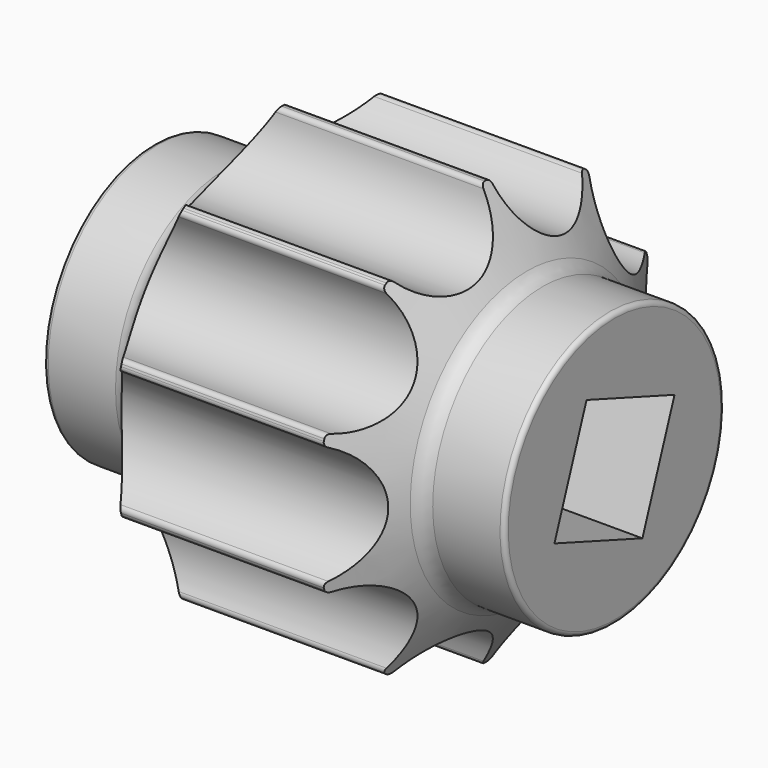
from build123d import *

# Parameters (mm, degrees)
F3_R        = 0.5
F2_R        = 5
F4_DEPTH    = 50
F2_R_2      = 7
F5_DEPTH    = 50
F6_R        = 2
F7_T1_DEPTH = 24.3069691613


# Not quite as in the source:
# - a fillet or chamfer that OpenCascade refuses, or shapes differently, is made with other operations: its cross-section is extruded or revolved along the edge and cut away or added
# - two fillets or chamfers of one size are made in one step


with BuildPart() as f1:
    # F0 (on Front) → F1 (revolve)
    with BuildSketch(Plane.XZ):
        Polygon((-25, 5), (25, 5), (25, 14.9), (16.1, 14.9), (11, 23), (-11, 23), (-16.1, 14.9), (-25, 14.9), align=None)
    revolve(axis=Axis((2.6108596474, 0, 0), (1, 0, 0)))

    # F3
    f3_edges = [f1.edges().sort_by_distance(p)[0] for p in [
        (-25, 0, -14.9),
        (25, 0, -14.9),
    ]]
    fillet(f3_edges, radius=F3_R)

    # F2 (on face) → F4 (cut)
    with BuildSketch(Plane.YZ.offset(25)):
        Polygon((3.7870547807, -8.1426786801), (8.1426786801, 3.7870547807), (-3.7870547807, 8.1426786801), (-8.1426786801, -3.7870547807), align=None)
        Circle(F2_R, mode=Mode.SUBTRACT)
    extrude(amount=-F4_DEPTH, mode=Mode.SUBTRACT)

    # F2 (on face) → F5 (cut)
    with BuildSketch(Plane.YZ.offset(25)):
        with Locations((19.8209163622, 14.4007386812)):
            Circle(F2_R_2)
        with Locations((24.5, 0)):
            Circle(F2_R_2)
        with Locations((19.8209163622, -14.4007386812)):
            Circle(F2_R_2)
        with Locations((7.5709163622, -23.3008846492)):
            Circle(F2_R_2)
        with Locations((-7.5709163622, -23.3008846492)):
            Circle(F2_R_2)
        with Locations((-19.8209163622, -14.4007386812)):
            Circle(F2_R_2)
        with Locations((-24.5, 0)):
            Circle(F2_R_2)
        with Locations((-7.5709163622, 23.3008846492)):
            Circle(F2_R_2)
        with Locations((7.5709163622, 23.3008846492)):
            Circle(F2_R_2)
        with Locations((-19.8209163622, 14.4007386812)):
            Circle(F2_R_2)
    extrude(amount=-F5_DEPTH, mode=Mode.SUBTRACT)

    # F6
    f6_edges = [f1.edges().sort_by_distance(p)[0] for p in [
        (-16.1, 0, -14.9),
        (16.1, 0, -14.9),
    ]]
    fillet(f6_edges, radius=F6_R)

    # F7: fillet of radius 0.5 on 20 edges, made by hand

    # F7_s2 → F7_t1 (cut)
    with BuildSketch(Plane.YZ.offset(-12.1534845806)):
        with BuildLine():
            ThreePointArc((12.7621083082, 18.6049793925), (13.0799593931, 18.7667461577), (13.424750127, 18.6755477571))
            ThreePointArc((13.424750127, 18.6755477571), (13.2367534387, 18.8092625693), (13.0474250079, 18.9410849917))
            ThreePointArc((13.0474250079, 18.9410849917), (12.9074134082, 18.7707853923), (12.7621083082, 18.6049793925))
        make_face()
        with BuildLine():
            ThreePointArc((0.1163605522, 22.9997056551), (0.4489071903, 22.8708238025), (0.6109700008, 22.5531235603))
            ThreePointArc((0.6109700008, 22.5531235603), (0.5908740269, 22.7726716267), (0.5777018563, 22.9927436502))
            ThreePointArc((0.5777018563, 22.9927436502), (0.3470486624, 22.9973815298), (0.1163605522, 22.9997056551))
        make_face()
        with BuildLine():
            ThreePointArc((-12.7621083082, 18.6049793925), (-13.0799593931, 18.7667461577), (-13.424750127, 18.6755477571))
            ThreePointArc((-13.424750127, 18.6755477571), (-13.2367534387, 18.8092625693), (-13.0474250079, 18.9410849917))
            ThreePointArc((-13.0474250079, 18.9410849917), (-12.9074134082, 18.7707853923), (-12.7621083082, 18.6049793925))
        make_face()
        with BuildLine():
            ThreePointArc((-0.1163605522, 22.9997056551), (-0.4489071903, 22.8708238025), (-0.6109700008, 22.5531235603))
            ThreePointArc((-0.6109700008, 22.5531235603), (-0.5908740269, 22.7726716267), (-0.5777018563, 22.9927436502))
            ThreePointArc((-0.5777018563, 22.9927436502), (-0.3470486624, 22.9973815298), (-0.1163605522, 22.9997056551))
        make_face()
        with BuildLine():
            ThreePointArc((13.6130254553, 18.5387577241), (13.8063064847, 18.2390241055), (13.7506785355, 17.8867410805))
            ThreePointArc((13.7506785355, 17.8867410805), (13.8634676667, 18.0761713143), (13.9821662468, 18.261955729))
            ThreePointArc((13.9821662468, 18.261955729), (13.7982899703, 18.4012823981), (13.6130254553, 18.5387577241))
        make_face()
        with BuildLine():
            ThreePointArc((21.2604950115, 7.5503654569), (21.6127260597, 7.4944093388), (21.8380625481, 7.2179653744))
            ThreePointArc((21.8380625481, 7.2179653744), (21.764565627, 7.4366446107), (21.6888789848, 7.6545756502))
            ThreePointArc((21.6888789848, 7.6545756502), (21.4755076282, 7.5990971335), (21.2604950115, 7.5503654569))
        make_face()
        with BuildLine():
            ThreePointArc((21.9099773243, 6.9966344517), (21.8901659611, 6.6405371218), (21.6380952381, 6.3882314559))
            ThreePointArc((21.6380952381, 6.3882314559), (21.8406878598, 6.4751879464), (22.0459183673, 6.5557214203))
            ThreePointArc((22.0459183673, 6.5557214203), (21.9790534962, 6.7765188269), (21.9099773243, 6.9966344517))
        make_face()
        with BuildLine():
            ThreePointArc((21.6380952381, -6.3882314559), (21.8901659611, -6.6405371218), (21.9099773243, -6.9966344517))
            ThreePointArc((21.9099773243, -6.9966344517), (21.9790534962, -6.7765188269), (22.0459183673, -6.5557214203))
            ThreePointArc((22.0459183673, -6.5557214203), (21.8406878598, -6.4751879464), (21.6380952381, -6.3882314559))
        make_face()
        with BuildLine():
            ThreePointArc((21.8380625481, -7.2179653744), (21.6127260597, -7.4944093388), (21.2604950115, -7.5503654569))
            ThreePointArc((21.2604950115, -7.5503654569), (21.4755076282, -7.5990971335), (21.6888789848, -7.6545756502))
            ThreePointArc((21.6888789848, -7.6545756502), (21.764565627, -7.4366446107), (21.8380625481, -7.2179653744))
        make_face()
        with BuildLine():
            ThreePointArc((13.7506785355, -17.8867410805), (13.8063064847, -18.2390241055), (13.6130254553, -18.5387577241))
            ThreePointArc((13.6130254553, -18.5387577241), (13.7982899703, -18.4012823981), (13.9821662468, -18.261955729))
            ThreePointArc((13.9821662468, -18.261955729), (13.8634676667, -18.0761713143), (13.7506785355, -17.8867410805))
        make_face()
        with BuildLine():
            ThreePointArc((13.424750127, -18.6755477571), (13.0799593931, -18.7667461577), (12.7621083082, -18.6049793925))
            ThreePointArc((12.7621083082, -18.6049793925), (12.9074134082, -18.7707853923), (13.0474250079, -18.9410849917))
            ThreePointArc((13.0474250079, -18.9410849917), (13.2367534387, -18.8092625693), (13.424750127, -18.6755477571))
        make_face()
        with BuildLine():
            ThreePointArc((0.1163605522, -22.9997056551), (0.4489071903, -22.8708238025), (0.6109700008, -22.5531235603))
            ThreePointArc((0.6109700008, -22.5531235603), (0.5908740269, -22.7726716267), (0.5777018563, -22.9927436502))
            ThreePointArc((0.5777018563, -22.9927436502), (0.3470486624, -22.9973815298), (0.1163605522, -22.9997056551))
        make_face()
        with BuildLine():
            ThreePointArc((-0.6109700008, -22.5531235603), (-0.4489071903, -22.8708238025), (-0.1163605522, -22.9997056551))
            ThreePointArc((-0.1163605522, -22.9997056551), (-0.3470486624, -22.9973815298), (-0.5777018563, -22.9927436502))
            ThreePointArc((-0.5777018563, -22.9927436502), (-0.5908740269, -22.7726716267), (-0.6109700008, -22.5531235603))
        make_face()
        with BuildLine():
            ThreePointArc((-13.424750127, -18.6755477571), (-13.0799593931, -18.7667461577), (-12.7621083082, -18.6049793925))
            ThreePointArc((-12.7621083082, -18.6049793925), (-12.9074134082, -18.7707853923), (-13.0474250079, -18.9410849917))
            ThreePointArc((-13.0474250079, -18.9410849917), (-13.2367534387, -18.8092625693), (-13.424750127, -18.6755477571))
        make_face()
        with BuildLine():
            ThreePointArc((-13.7506785355, -17.8867410805), (-13.8063064847, -18.2390241055), (-13.6130254553, -18.5387577241))
            ThreePointArc((-13.6130254553, -18.5387577241), (-13.7982899703, -18.4012823981), (-13.9821662468, -18.261955729))
            ThreePointArc((-13.9821662468, -18.261955729), (-13.8634676667, -18.0761713143), (-13.7506785355, -17.8867410805))
        make_face()
        with BuildLine():
            ThreePointArc((-21.8380625481, -7.2179653744), (-21.6127260597, -7.4944093388), (-21.2604950115, -7.5503654569))
            ThreePointArc((-21.2604950115, -7.5503654569), (-21.4755076282, -7.5990971335), (-21.6888789848, -7.6545756502))
            ThreePointArc((-21.6888789848, -7.6545756502), (-21.764565627, -7.4366446107), (-21.8380625481, -7.2179653744))
        make_face()
        with BuildLine():
            ThreePointArc((-21.6380952381, -6.3882314559), (-21.8901659611, -6.6405371218), (-21.9099773243, -6.9966344517))
            ThreePointArc((-21.9099773243, -6.9966344517), (-21.9790534962, -6.7765188269), (-22.0459183673, -6.5557214203))
            ThreePointArc((-22.0459183673, -6.5557214203), (-21.8406878598, -6.4751879464), (-21.6380952381, -6.3882314559))
        make_face()
        with BuildLine():
            ThreePointArc((-21.9099773243, 6.9966344517), (-21.8901659611, 6.6405371218), (-21.6380952381, 6.3882314559))
            ThreePointArc((-21.6380952381, 6.3882314559), (-21.8406878598, 6.4751879464), (-22.0459183673, 6.5557214203))
            ThreePointArc((-22.0459183673, 6.5557214203), (-21.9790534962, 6.7765188269), (-21.9099773243, 6.9966344517))
        make_face()
        with BuildLine():
            ThreePointArc((-21.2604950115, 7.5503654569), (-21.6127260597, 7.4944093388), (-21.8380625481, 7.2179653744))
            ThreePointArc((-21.8380625481, 7.2179653744), (-21.764565627, 7.4366446107), (-21.6888789848, 7.6545756502))
            ThreePointArc((-21.6888789848, 7.6545756502), (-21.4755076282, 7.5990971335), (-21.2604950115, 7.5503654569))
        make_face()
        with BuildLine():
            ThreePointArc((-13.6130254553, 18.5387577241), (-13.8063064847, 18.2390241055), (-13.7506785355, 17.8867410805))
            ThreePointArc((-13.7506785355, 17.8867410805), (-13.8634676667, 18.0761713143), (-13.9821662468, 18.261955729))
            ThreePointArc((-13.9821662468, 18.261955729), (-13.7982899703, 18.4012823981), (-13.6130254553, 18.5387577241))
        make_face()
    extrude(amount=F7_T1_DEPTH, mode=Mode.SUBTRACT)


with BuildPart() as f9_1:
    # F9: copy of F1
    add(f1.part.moved(Location((0, 71.6, 0))))


solid = f1.part
